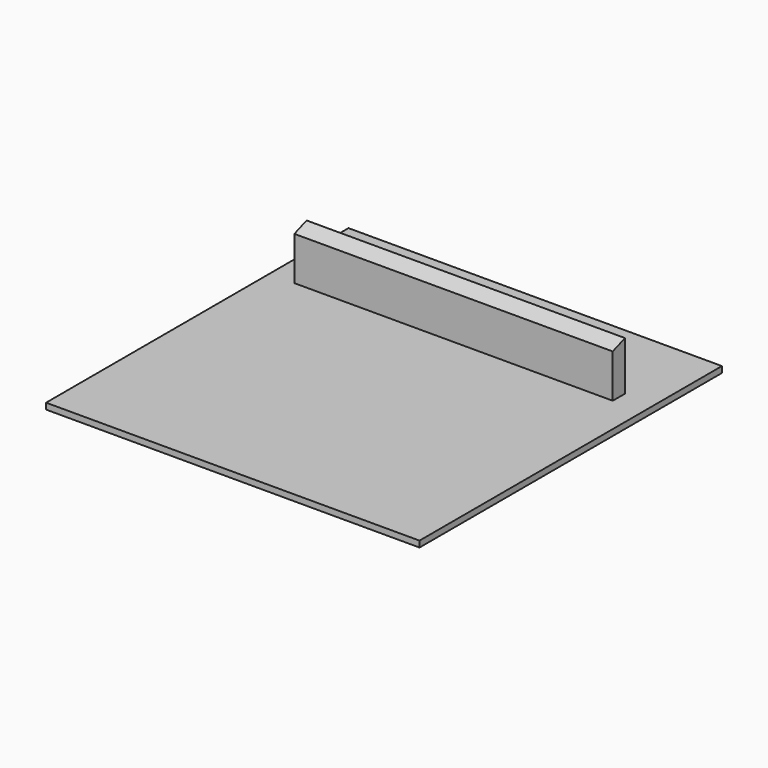
from build123d import *

# Parameters (mm, degrees)
F0_W     = 104.0173918009
F0_H     = 5
F1_DEPTH = 2
F2_DEPTH = 16
F3_SIZE2 = 1.819841
F3_SIZE  = 4.99999


# Not quite as in the source:
# - a fillet or chamfer is up to 0.001 mm smaller than in the source, because OpenCascade refuses the exact size


with BuildPart() as f1:
    # F0 (on Top) → F1 (new body)
    with BuildSketch(Plane.XY):
        Polygon((-72.627124867, 48.6539505273), (-75.627124867, 48.6539505273), (-75.627124867, -74.8460494727), (-72.627124867, -74.8460494727), (-14.627124867, -74.8460494727), (-14.3716531694, -74.8460494727), (43.372875133, -74.8460494727), (46.372875133, -74.8460494727), (46.372875133, 48.6539505273), (43.372875133, 48.6539505273), (-14.3716531694, 48.6539505273), (-14.627124867, 48.6539505273), (-14.8716531694, 48.6539505273), align=None)
        with Locations((-15.4112055898, 18.7856731331)):
            Rectangle(F0_W, F0_H, mode=Mode.SUBTRACT)
        with Locations((-15.4112055898, 18.7856731331)):
            Rectangle(F0_W, F0_H)
    extrude(amount=-F1_DEPTH)

    # F0 (on Top) → F2 (join)
    with BuildSketch(Plane.XY):
        with Locations((-15.4112055898, 18.7856731331)):
            Rectangle(F0_W, F0_H)
    extrude(amount=F2_DEPTH)

    # F3 (size 5 and 1.8198511713 in the source; OpenCascade refuses exactly that, so slightly less here)
    f3_edges = [f1.edges().sort_by_distance(p)[0] for p in [
        (-15.411206, 16.285673, 16),
    ]]
    f3_side = f1.faces().sort_by_distance((-15.411206, 18.785673, 16))[0]
    chamfer(f3_edges, length=F3_SIZE, length2=F3_SIZE2, reference=f3_side)


solid = f1.part
